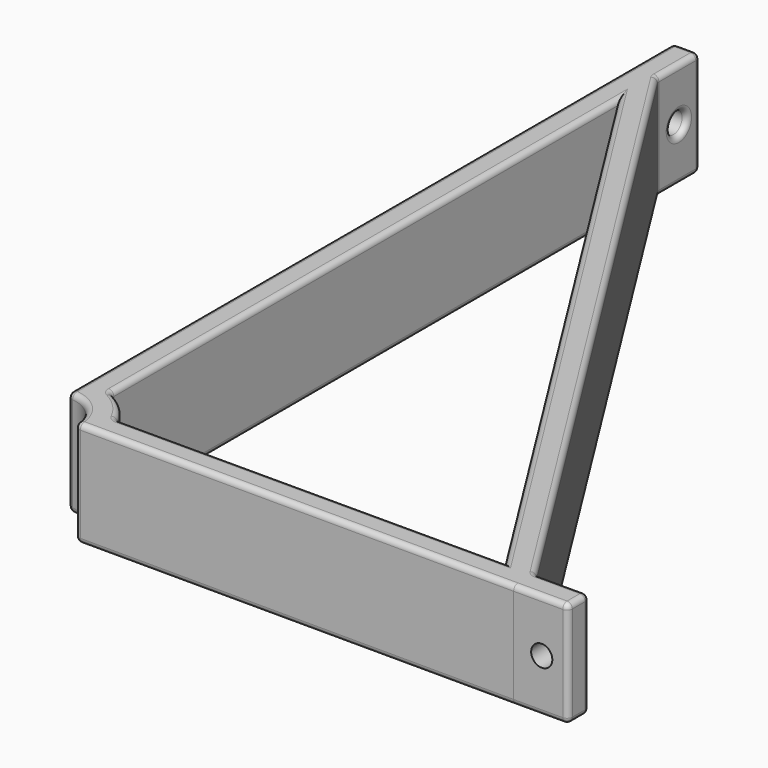
from build123d import *

# Parameters (mm, degrees)
F1_DEPTH = 20
F2_R     = 2
F3_DEPTH = 25
F4_R     = 2
F5_DEPTH = 25
F6_R     = 1


# Not quite as in the source:
# - a feature names something its author has since deleted; it is built from what else it names


with BuildPart() as f1:
    # F0 (on Top) → F1 (new body)
    with BuildSketch(Plane.XY):
        Polygon((84.3844267085, 4.7044013627), (90.2951131996, 4.7044013627), (5, 140), (5, 130.6244351268), align=None)
        with BuildLine():
            Line((100.2951131996, 4.7044013627), (90.2951131996, 4.7044013627))
            Line((90.2951131996, 4.7044013627), (84.3844267085, 4.7044013627))
            Line((84.3844267085, 4.7044013627), (10.95945259, 4.7044013627))
            ThreePointArc((10.95945259, 4.7044013627), (8.5469291421, 8.3181124958), (5, 10.8277880129))
            Line((5, 10.8277880129), (5, 130.6244351268))
            Line((5, 130.6244351268), (5, 140))
            Line((5, 140), (5, 150))
            Line((5, 150), (0, 150))
            Line((0, 150), (0, 6.9264828534))
            ThreePointArc((0, 6.9264828534), (4.9057995801, 4.8897132021), (6.9264454937, -0.0227495433))
            Line((6.9264454937, -0.0227495433), (89.9995145623, -0.2955986373))
            Line((89.9995145623, -0.2955986373), (100.2951131996, -0.2955986373))
            Line((100.2951131996, -0.2955986373), (100.2951131996, 4.7044013627))
        make_face()
    extrude(amount=F1_DEPTH)

    # F2 (on face) → F3 (cut)
    with BuildSketch(Plane.YZ.offset(5)):
        with Locations((145, 10)):
            Circle(F2_R)
    extrude(amount=-F3_DEPTH, mode=Mode.SUBTRACT)

    # F4 (on face) → F5 (cut)
    with BuildSketch(Plane(origin=(0, 4.7044013627, 0), x_dir=(-1, 0, 0), z_dir=(0, 1, 0))):
        with Locations((-95.3095704317, 10)):
            Circle(F4_R)
    extrude(amount=-F5_DEPTH, mode=Mode.SUBTRACT)

    # F6
    f6_edges = [f1.edges().sort_by_distance(p)[0] for p in [
        (100.295113, 4.704401, 10),
        (47.647557, 72.352201, 20),
        (5, 145, 20),
        (2.5, 150, 20),
        (0, 78.463241, 20),
        (4.9058, 4.889713, 20),
        (48.46298, -0.159174, 20),
        (95.147314, -0.295599, 20),
        (100.295113, 2.204401, 20),
        (95.295113, 4.704401, 20),
        (44.692213, 67.664418, 20),
        (47.67194, 4.704401, 20),
        (8.546929, 8.318112, 20),
        (5, 70.726112, 20),
        (47.647557, 72.352201, 0),
        (5, 145, 0),
        (2.5, 150, 0),
        (0, 78.463241, 0),
        (4.9058, 4.889713, 0),
        (48.46298, -0.159174, 0),
        (95.147314, -0.295599, 0),
        (100.295113, 2.204401, 0),
        (95.295113, 4.704401, 0),
        (44.692213, 67.664418, 0),
        (47.67194, 4.704401, 0),
        (8.546929, 8.318112, 0),
        (5, 70.726112, 0),
        (5, 143, 10),
        (97.30957, 4.704401, 10),
        (90.295113, 4.704401, 10),
        (5, 140, 10),
        (5, 150, 10),
        (6.926445, -0.02275, 10),
        (0, 6.926483, 10),
        (5, 10.827788, 10),
        (10.959453, 4.704401, 10),
        (100.295113, -0.295599, 10),
        (0, 150, 10),
    ]]
    fillet(f6_edges, radius=F6_R)


solid = f1.part
